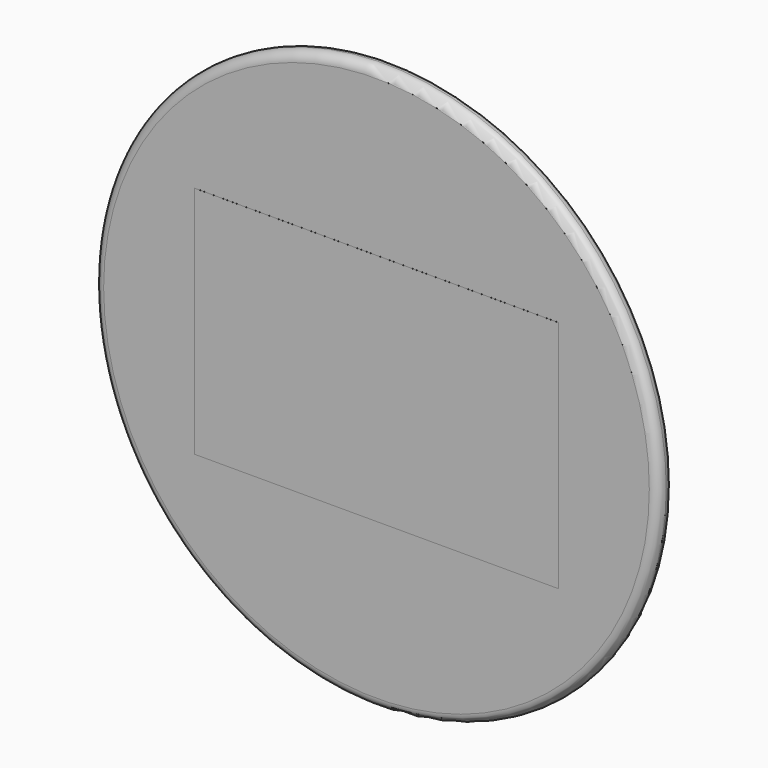
from build123d import *

# Parameters (mm, degrees)
F0_R     = 152.4
F0_W     = 196.5556636505
F0_H     = 126.4792977641
F1_DEPTH = 5.08
F3_R     = 5.07999
F4_DEPTH = 5.08
F5_W     = 196.5556636505
F5_H     = 126.4792977641
F6_DEPTH = 0.0254


# Not quite as in the source:
# - a fillet or chamfer is up to 0.001 mm smaller than in the source, because OpenCascade refuses the exact size
# - the program builds the solid bodies; features that only make, move or delete a surface that nothing else refers to are left out


with BuildPart() as f1:
    # F0 (on Front) → F1 (new body, symmetric)
    with BuildSketch(Plane.XZ):
        Circle(F0_R)
        Rectangle(F0_W, F0_H, mode=Mode.SUBTRACT)
    extrude(amount=F1_DEPTH, both=True)

    # F3 (radius 5.08 in the source; OpenCascade refuses exactly that, so slightly less here)
    f3_edges = [f1.edges().sort_by_distance(p)[0] for p in [
        (-152.4, 5.08, 0),
        (-152.4, -5.08, 0),
    ]]
    fillet(f3_edges, radius=F3_R)

    # F0 (on Front) → F4 (join)
    with BuildSketch(Plane.XZ):
        Rectangle(F0_W, F0_H)
    extrude(amount=-F4_DEPTH)


with BuildPart() as f6:
    # F5 (on face) → F6 (new body)
    with BuildSketch(Plane.XZ.offset(5.08)):
        Rectangle(F5_W, F5_H)
    extrude(amount=F6_DEPTH)


solid = Compound([f1.part, f6.part])
